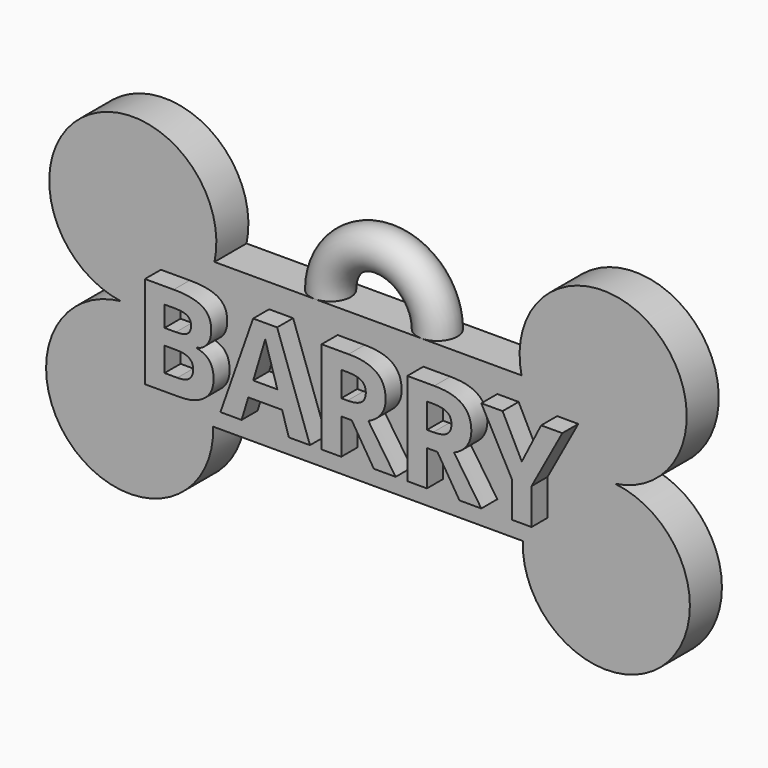
from build123d import *

# Parameters (mm, degrees)
F2_DEPTH     = 3
F0_TEXT_SIZE = 9.7222222222
F3_DEPTH     = 1.5


# Not quite as in the source:
# - Text() gives the source's letters only with a copy of the font that has no kerning and outlines rounded to 1/6400 em; it was checked with that copy


with BuildPart() as f2:
    # F1 (on Front) → F2 (new body)
    with BuildSketch(Plane.XZ):
        with BuildLine():
            Line((9.7992818472, 5.758833701), (-13.2007181528, 5.758833701))
            ThreePointArc((-13.2007181528, 5.758833701), (-22.8919967583, 12.2303025958), (-20.2068222461, 0.8905217996))
            ThreePointArc((-20.2068222461, 0.8905217996), (-23.6694108068, -10.0559002963), (-13.2974652522, -5.1328502605))
            Line((-13.2974652522, -5.1328502605), (9.8960289467, -5.1328502605))
            ThreePointArc((9.8960289467, -5.1328502605), (20.2679745012, -10.0559002963), (16.8053859406, 0.8905217996))
            ThreePointArc((16.8053859406, 0.8905217996), (19.4905604528, 12.2303025958), (9.7992818472, 5.758833701))
        make_face()
    extrude(amount=-F2_DEPTH)

    # F5 (on 3pt) → F6 (revolve)
    with BuildSketch(Plane.XY.offset(5.758833701)):
        with BuildLine():
            ThreePointArc((0.7992818472, 1.5), (2.2992818472, 0), (3.7992818472, 1.5))
            ThreePointArc((3.7992818472, 1.5), (2.2992818472, 3), (0.7992818472, 1.5))
        make_face()
    revolve(axis=Axis((-1.7007181528, 1.5, 5.758833701), (0, 1, 0)))


with BuildPart() as f3:
    # F0 (on Front) → F3 (new body)
    with BuildSketch(Plane.XZ):
        with Locations((-18.0879794375, -3)):
            Text('BARRY', F0_TEXT_SIZE, font='Open Sans', font_style=FontStyle.BOLD, text_align=(TextAlign.LEFT, TextAlign.BOTTOM))
    extrude(amount=F3_DEPTH)


solid = Compound([f2.part, f3.part])
